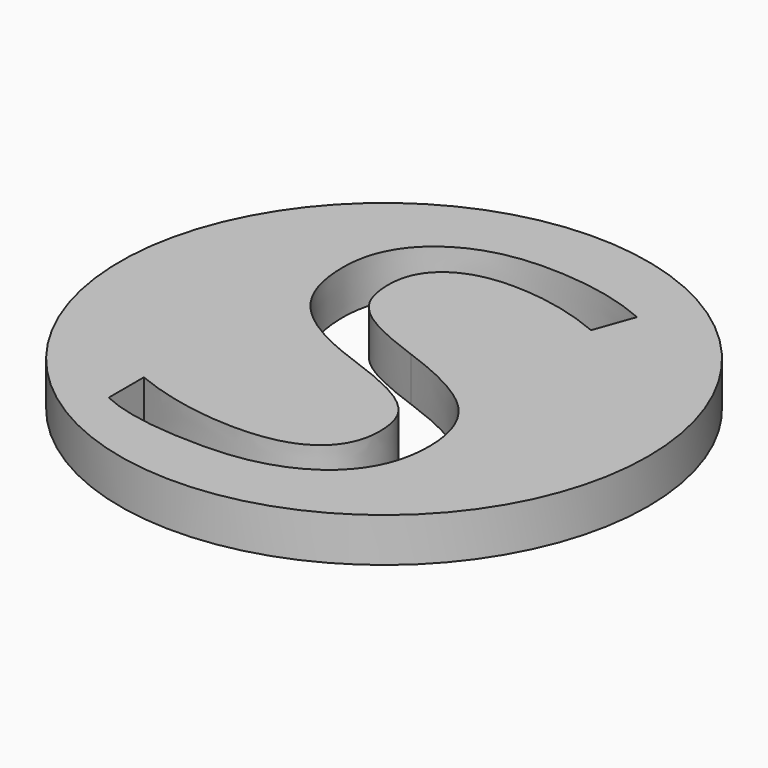
from build123d import *

# Parameters (mm, degrees)
F0_R         = 12
F1_DEPTH     = 2
F2_TEXT_SIZE = 25
F3_DEPTH     = 25


# Not quite as in the source:
# - Text() gives the source's letters only with a copy of the font that has no kerning and outlines rounded to 1/6400 em; it was checked with that copy


with BuildPart() as f1:
    # F0 (on Top) → F1 (new body)
    with BuildSketch(Plane.XY):
        Circle(F0_R)
    extrude(amount=F1_DEPTH)

    # F2 (on face) → F3 (cut)
    with BuildSketch(Plane.XY.offset(2)):
        with Locations((-7.072265625, -9)):
            Text('S', F2_TEXT_SIZE, font='Open Sans', text_align=(TextAlign.LEFT, TextAlign.BOTTOM))
    extrude(amount=-F3_DEPTH, mode=Mode.SUBTRACT)


solid = f1.part
